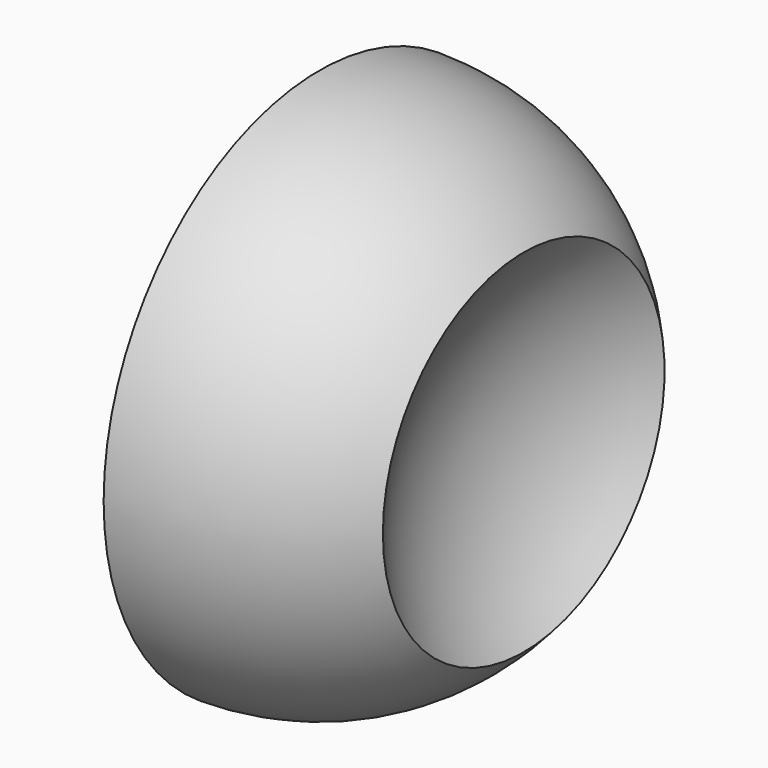
from build123d import *


# Not quite as in the source:
# - a feature names something its author has since deleted; it is built from what else it names


with BuildPart() as f1:
    # F0 (on Top) → F1 (revolve)
    with BuildSketch(Plane.XY):
        with BuildLine():
            ThreePointArc((46.04, -43.0037021662), (26.4665845911, -57.1709707813), (3, -62.9285308902))
            Line((3, -62.9285308902), (3, 0))
            Line((3, 0), (0, 0))
            Line((0, 0), (0, -66))
            ThreePointArc((0, -66), (27.5012088992, -59.9973625177), (50, -43.0813184571))
            ThreePointArc((50, -43.0813184571), (38.129166807, -22.9782505862), (34, 0))
            Line((34, 0), (31, 0))
            ThreePointArc((31, 0), (34.8684408293, -22.7789376398), (46.04, -43.0037021662))
        make_face()
    revolve(axis=Axis((-14.5, 0, 0), (-1, 0, 0)))


solid = f1.part
